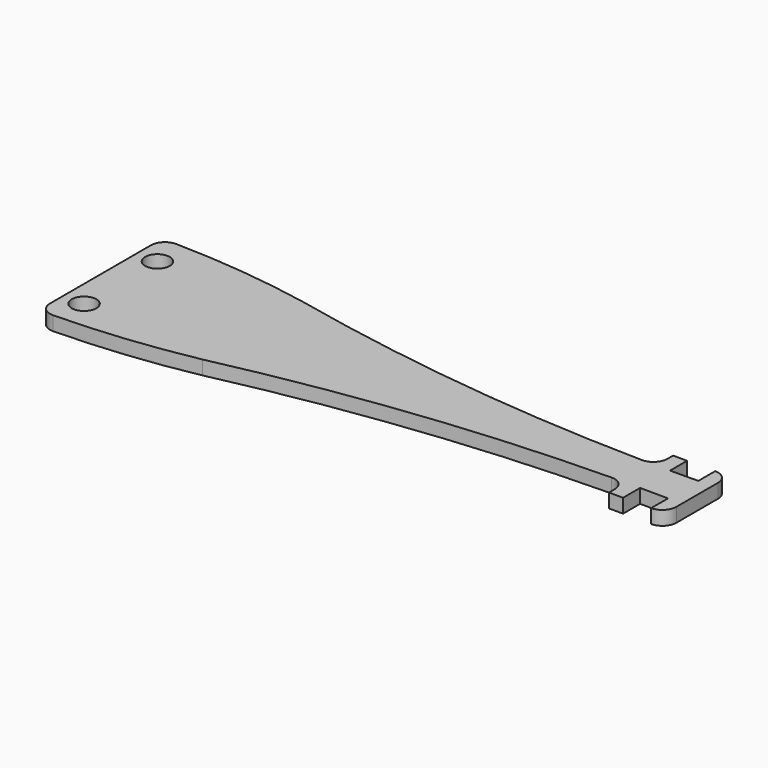
from build123d import *

# Parameters (mm, degrees)
F0_R     = 1.75
F1_DEPTH = 2
F2_R     = 1.99999


# Not quite as in the source:
# - a fillet or chamfer is up to 0.001 mm smaller than in the source, because OpenCascade refuses the exact size


with BuildPart() as f1:
    # F0 (on Top) → F1 (new body)
    with BuildSketch(Plane.XY):
        with BuildLine():
            Line((0, 22), (0, 0))
            ThreePointArc((0, 0), (10.8792490031, 0.5215994991), (21.6586962342, 2.0816130564))
            ThreePointArc((21.6586962342, 2.0816130564), (49.1649189112, 6.6602813892), (77, 8.3230352611))
            ThreePointArc((77, 8.3230352611), (77.9999938672, 8.3281723489), (79, 8.3295355292))
            ThreePointArc((79, 8.3295355292), (81.0000609284, 8.3209395881), (83, 8.2972474438))
            ThreePointArc((83, 8.2972474438), (84.0000366078, 8.2797378058), (85, 8.2584535703))
            Line((85, 8.2584535703), (85, 13.7415464297))
            ThreePointArc((85, 13.7415464297), (84.0000366078, 13.7202621942), (83, 13.7027525562))
            ThreePointArc((83, 13.7027525562), (81.0000609284, 13.6790604119), (79, 13.6704644708))
            ThreePointArc((79, 13.6704644708), (77.9999938672, 13.6718276511), (77, 13.6769647389))
            ThreePointArc((77, 13.6769647389), (49.1649189112, 15.3397186108), (21.6586962342, 19.9183869436))
            ThreePointArc((21.6586962342, 19.9183869436), (10.8792490031, 21.4784005009), (0, 22))
        make_face()
        with Locations((3, 4.3338485993)):
            Circle(F0_R, mode=Mode.SUBTRACT)
        with Locations((3, 17.3932574689)):
            Circle(F0_R, mode=Mode.SUBTRACT)
        with BuildLine():
            ThreePointArc((79, 8.3295355292), (77.9999938672, 8.3281723489), (77, 8.3230352611))
            Line((77, 8.3230352611), (77, 5.2972474438))
            Line((77, 5.2972474438), (79, 5.2972474438))
            Line((79, 5.2972474438), (79, 8.3295355292))
        make_face()
        with BuildLine():
            Line((83, 5.2972474438), (85, 5.2972474438))
            Line((85, 5.2972474438), (85, 8.2584535703))
            ThreePointArc((85, 8.2584535703), (84.0000366078, 8.2797378058), (83, 8.2972474438))
            Line((83, 8.2972474438), (83, 5.2972474438))
        make_face()
        with BuildLine():
            Line((77, 16.7027525562), (77, 13.6769647389))
            ThreePointArc((77, 13.6769647389), (77.9999938672, 13.6718276511), (79, 13.6704644708))
            Line((79, 13.6704644708), (79, 16.7027525562))
            Line((79, 16.7027525562), (77, 16.7027525562))
        make_face()
        with BuildLine():
            Line((85, 13.7415464297), (85, 16.7027525562))
            Line((85, 16.7027525562), (83, 16.7027525562))
            Line((83, 16.7027525562), (83, 13.7027525562))
            ThreePointArc((83, 13.7027525562), (84.0000366078, 13.7202621942), (85, 13.7415464297))
        make_face()
    extrude(amount=F1_DEPTH)

    # F2 (radius 2 in the source; OpenCascade refuses exactly that, so slightly less here)
    f2_edges = [f1.edges().sort_by_distance(p)[0] for p in [
        (0, 0, 1),
        (0, 22, 1),
        (85, 5.297247, 1),
        (85, 16.702753, 1),
        (77, 8.323035, 1),
        (77, 13.676965, 1),
    ]]
    fillet(f2_edges, radius=F2_R)


solid = f1.part
